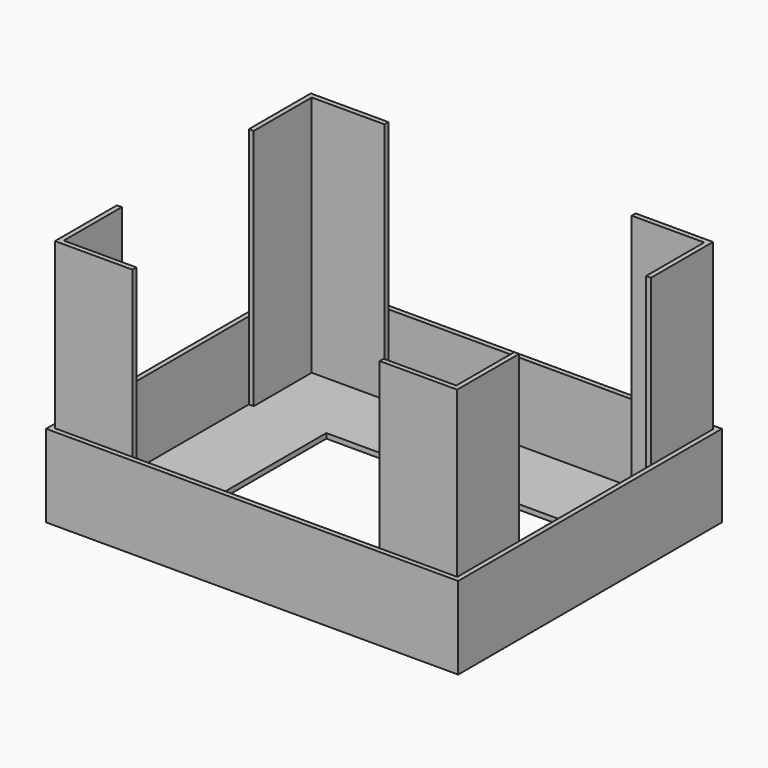
from build123d import *

# Parameters (mm, degrees)
F1_DEPTH = 150
F2_DEPTH = 150
F3_DEPTH = 50
F0_W     = 44.041014101
F0_H     = 44.0000000126
F4_DEPTH = 3


# Not quite as in the source:
# - ends of sketch curves that miss each other by under 0.0002 mm in the source are joined


with BuildPart() as f1:
    # F0 (on Top) → F1 (new body)
    with BuildSketch(Plane.XY):
        Polygon((-133.6856555302, 90.2236848028), (-89.6446414292, 90.2236848154), (-89.6446414292, 93.2236848154), (-136.6471022147, 93.2236848019), (-136.6471022147, 46.2236531798), (-133.6856555302, 46.2212240181), align=None)
    extrude(amount=F1_DEPTH)


with BuildPart() as f2:
    # F0 (on Top) → F2 (new body)
    with BuildSketch(Plane.XY):
        Polygon((60.3553585708, 93.2236848154), (60.3553585708, 90.2236848154), (104.3963726718, 90.2236848028), (104.3963726718, 46.2212240181), (107.3578193563, 46.2236531798), (107.3578193563, 93.2236848019), align=None)
    extrude(amount=F2_DEPTH)


with BuildPart() as f2b:
    # F0 (on Top) → F2, piece 2 (new body)
    with BuildSketch(Plane.XY):
        Polygon((107.3578193563, -53.7763151981), (104.3963726718, -53.7763151981), (104.3963726718, -97.7763151981), (60.3553585708, -97.7763152106), (60.3553585708, -100.7763152106), (107.3578193563, -100.7763151981), (107.3963716626, -53.7763151981), align=None)
    extrude(amount=F2_DEPTH)


with BuildPart() as f2c:
    # F0 (on Top) → F2, piece 3 (new body)
    with BuildSketch(Plane.XY):
        Polygon((-89.6446414292, -100.7763152106), (-89.6446414292, -97.7763152106), (-133.6856555302, -97.7763151981), (-133.6856555302, -53.7763151981), (-136.6471022147, -53.7763151981), (-136.6471022147, -100.7763151981), align=None)
    extrude(amount=F2_DEPTH)


with BuildPart() as f3:
    # F0 (on Top) → F3 (new body)
    with BuildSketch(Plane.XY):
        Polygon((-89.6446414292, 96.2236848019), (-136.6446414292, 96.2236848019), (-139.6446414292, 96.2236848019), (-139.6446414292, 46.2236848019), (-139.6446414292, -3.7763151976), (-139.6446414292, -103.7763151981), (110.3553585708, -103.7763151981), (110.3553585708, -53.7763151981), (110.3553585708, 96.2236848019), (60.3553585708, 96.2236848019), (-14.6446414292, 96.2236848019), align=None)
        Polygon((-136.6471022147, 93.2236848019), (-89.6446414292, 93.2236848154), (60.3553585708, 93.2236848154), (107.3578193563, 93.2236848019), (107.3963716626, 46.2236848019), (107.3963716626, -53.7763151981), (107.3963716626, -100.7763151981), (107.3578193563, -100.7763151981), (60.3553585708, -100.7763151981), (-89.6446414292, -100.7763151981), (-136.6471022147, -100.7763151981), (-136.685654521, -53.7763151981), (-136.685654521, 46.2236848028), align=None, mode=Mode.SUBTRACT)
    extrude(amount=F3_DEPTH)


with BuildPart() as f4:
    # F0 (on Top) → F4 (new body)
    with BuildSketch(Plane.XY):
        with Locations((-111.6651484797, -75.7763152043)):
            Rectangle(F0_W, F0_H)
        Polygon((-89.6446414292, -53.7763151981), (-89.6446414292, 46.2236848019), (-89.6446414292, 90.2236848154), (-133.6856555302, 90.2236848028), (-133.6856555302, 46.2212240181), (-136.6471022147, 46.2236531798), (-136.6471022147, -53.7763151981), (-133.6856555302, -53.7738544134), (-133.6856555302, -53.7763151981), align=None)
        Polygon((60.3553585708, -53.7763151981), (-89.6446414292, -53.7763151981), (-89.6446414292, -97.7763152106), (-89.6446414292, -100.7763152106), (60.3553585708, -100.7763151981), (60.3553585708, -97.7763152106), (104.3963726718, -97.7763151981), (104.3963726718, -53.7763151981), align=None)
        Polygon((60.3553585708, 90.2236848154), (60.3553585708, 46.2236848019), (60.3553585708, -53.7763151981), (104.3963726718, -53.7763151981), (104.3963726718, -53.7738544134), (107.3578193823, -53.7762835751), (107.3963716626, -53.7763151981), (107.3963716626, 46.2236848019), (107.3578193563, 46.2236531798), (104.3963726718, 46.2212240181), (104.3963726718, 90.2236848028), align=None)
        Polygon((-89.6446414292, 90.2236848154), (-89.6446414292, 46.2236848019), (60.3553585708, 46.2236848019), (60.3553585708, 90.2236848154), (60.3553585708, 93.2236848154), (-89.6446414292, 93.2236848154), align=None)
    extrude(amount=F4_DEPTH)


solid = Compound([f1.part, f2.part, f2b.part, f2c.part, f3.part, f4.part])
